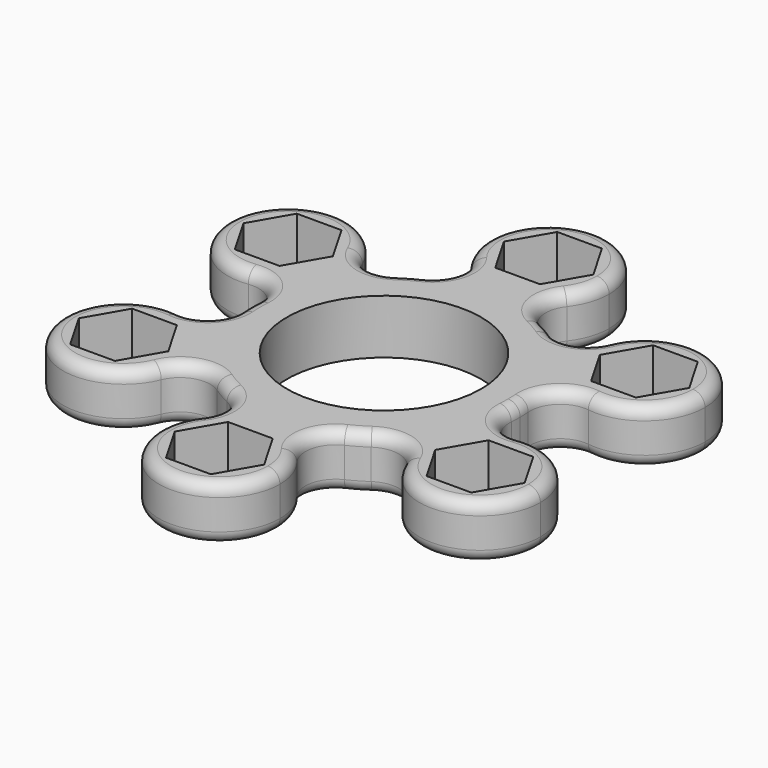
from build123d import *

# Parameters (mm, degrees)
F0_R     = 16.05
F1_DEPTH = 9
F2_R     = 2


# Not quite as in the source:
# - a feature names something its author has since deleted; it is built from what else it names


with BuildPart() as f1:
    # F0 (on Top) → F1 (new body)
    with BuildSketch(Plane.XY):
        with BuildLine():
            ThreePointArc((22.4319147865, -1.749056606), (22.4829722534, -0.8751906374), (22.5, 0))
            ThreePointArc((22.5, 0), (22.4829722534, 0.8751906374), (22.4319147865, 1.749056606))
            ThreePointArc((22.4319147865, 1.749056606), (19.4855715851, 11.25), (12.7306848467, 18.5520797576))
            ThreePointArc((12.7306848467, 18.5520797576), (11.25, 19.4855715851), (9.7012299398, 20.3011363636))
            ThreePointArc((9.7012299398, 20.3011363636), (0, 22.5), (-9.7012299398, 20.3011363636))
            ThreePointArc((-9.7012299398, 20.3011363636), (-11.25, 19.4855715851), (-12.7306848467, 18.5520797576))
            ThreePointArc((-12.7306848467, 18.5520797576), (-19.4855715851, 11.25), (-22.4319147865, 1.749056606))
            ThreePointArc((-22.4319147865, 1.749056606), (-22.5, 0), (-22.4319147865, -1.749056606))
            ThreePointArc((-22.4319147865, -1.749056606), (-19.4855715851, -11.25), (-12.7306848467, -18.5520797576))
            ThreePointArc((-12.7306848467, -18.5520797576), (-11.25, -19.4855715851), (-9.7012299398, -20.3011363636))
            ThreePointArc((-9.7012299398, -20.3011363636), (0, -22.5), (9.7012299398, -20.3011363636))
            ThreePointArc((9.7012299398, -20.3011363636), (11.25, -19.4855715851), (12.7306848467, -18.5520797576))
            ThreePointArc((12.7306848467, -18.5520797576), (19.4855715851, -11.25), (22.4319147865, -1.749056606))
        make_face()
        Circle(F0_R, mode=Mode.SUBTRACT)
        with BuildLine():
            ThreePointArc((12.7306848467, 18.5520797576), (19.4855715851, 11.25), (22.4319147865, 1.749056606))
            ThreePointArc((22.4319147865, 1.749056606), (23.9849013008, 5.7739668766), (28.0928110689, 7.0918239012))
            ThreePointArc((28.0928110689, 7.0918239012), (20.7846096908, 12), (20.1881051921, 20.7831760988))
            ThreePointArc((20.1881051921, 20.7831760988), (16.9928526462, 17.8845503954), (12.7306848467, 18.5520797576))
        make_face()
        with BuildLine():
            ThreePointArc((28.0928110689, -7.0918239012), (23.9849013008, -5.7739668766), (22.4319147865, -1.749056606))
            ThreePointArc((22.4319147865, -1.749056606), (19.4855715851, -11.25), (12.7306848467, -18.5520797576))
            ThreePointArc((12.7306848467, -18.5520797576), (16.9928526462, -17.8845503954), (20.1881051921, -20.7831760988))
            ThreePointArc((20.1881051921, -20.7831760988), (20.7846096908, -12), (28.0928110689, -7.0918239012))
        make_face()
        with BuildLine():
            ThreePointArc((20.1881051921, 20.7831760988), (20.7846096908, 12), (28.0928110689, 7.0918239012))
            ThreePointArc((28.0928110689, 7.0918239012), (36.0205565972, 9.4660592451), (39.4448637287, 17))
            ThreePointArc((39.4448637287, 17), (31.3726104228, 26.8124305186), (20.1881051921, 20.7831760988))
        make_face()
        Polygon((36.8349471743, 17), (33.1399054515, 10.6), (25.7498220059, 10.6), (22.054780283, 17), (25.7498220059, 23.4), (33.1399054515, 23.4), align=None, mode=Mode.SUBTRACT)
        with BuildLine():
            ThreePointArc((39.4448637287, -17), (36.0205565972, -9.4660592451), (28.0928110689, -7.0918239012))
            ThreePointArc((28.0928110689, -7.0918239012), (20.7846096908, -12), (20.1881051921, -20.7831760988))
            ThreePointArc((20.1881051921, -20.7831760988), (31.3726104228, -26.8124305186), (39.4448637287, -17))
        make_face()
        Polygon((22.054780283, -17), (25.7498220059, -10.6), (33.1399054515, -10.6), (36.8349471743, -17), (33.1399054515, -23.4), (25.7498220059, -23.4), align=None, mode=Mode.SUBTRACT)
        with BuildLine():
            ThreePointArc((-9.7012299398, 20.3011363636), (0, 22.5), (9.7012299398, 20.3011363636))
            ThreePointArc((9.7012299398, 20.3011363636), (6.9920486546, 23.6585172721), (7.9047058769, 27.875))
            ThreePointArc((7.9047058769, 27.875), (0, 24), (-7.9047058769, 27.875))
            ThreePointArc((-7.9047058769, 27.875), (-6.9920486546, 23.6585172721), (-9.7012299398, 20.3011363636))
        make_face()
        with BuildLine():
            ThreePointArc((7.9047058769, -27.875), (6.9920486546, -23.6585172721), (9.7012299398, -20.3011363636))
            ThreePointArc((9.7012299398, -20.3011363636), (0, -22.5), (-9.7012299398, -20.3011363636))
            ThreePointArc((-9.7012299398, -20.3011363636), (-6.9920486546, -23.6585172721), (-7.9047058769, -27.875))
            ThreePointArc((-7.9047058769, -27.875), (0, -24), (7.9047058769, -27.875))
        make_face()
        with BuildLine():
            ThreePointArc((-7.9047058769, 27.875), (0, 24), (7.9047058769, 27.875))
            ThreePointArc((7.9047058769, 27.875), (9.4616874491, 30.7632623499), (10, 34))
            ThreePointArc((10, 34), (-3.2367376501, 43.4616874491), (-7.9047058769, 27.875))
        make_face()
        Polygon((7.3900834456, 34), (3.6950417228, 27.6), (-3.6950417228, 27.6), (-7.3900834456, 34), (-3.6950417228, 40.4), (3.6950417228, 40.4), align=None, mode=Mode.SUBTRACT)
        with BuildLine():
            ThreePointArc((10, -34), (9.4616874491, -30.7632623499), (7.9047058769, -27.875))
            ThreePointArc((7.9047058769, -27.875), (0, -24), (-7.9047058769, -27.875))
            ThreePointArc((-7.9047058769, -27.875), (-3.2367376501, -43.4616874491), (10, -34))
        make_face()
        Polygon((-7.3900834456, -34), (-3.6950417228, -27.6), (3.6950417228, -27.6), (7.3900834456, -34), (3.6950417228, -40.4), (-3.6950417228, -40.4), align=None, mode=Mode.SUBTRACT)
        with BuildLine():
            ThreePointArc((-22.4319147865, 1.749056606), (-19.4855715851, 11.25), (-12.7306848467, 18.5520797576))
            ThreePointArc((-12.7306848467, 18.5520797576), (-16.9928526462, 17.8845503954), (-20.1881051921, 20.7831760988))
            ThreePointArc((-20.1881051921, 20.7831760988), (-19.63243321, 18.9277466942), (-19.4448637287, 17))
            ThreePointArc((-19.4448637287, 17), (-21.9109229737, 10.4243071315), (-28.0928110689, 7.0918239012))
            ThreePointArc((-28.0928110689, 7.0918239012), (-23.9849013008, 5.7739668766), (-22.4319147865, 1.749056606))
        make_face()
        with BuildLine():
            ThreePointArc((-20.1881051921, -20.7831760988), (-16.9928526462, -17.8845503954), (-12.7306848467, -18.5520797576))
            ThreePointArc((-12.7306848467, -18.5520797576), (-19.4855715851, -11.25), (-22.4319147865, -1.749056606))
            ThreePointArc((-22.4319147865, -1.749056606), (-23.9849013008, -5.7739668766), (-28.0928110689, -7.0918239012))
            ThreePointArc((-28.0928110689, -7.0918239012), (-21.9109229737, -10.4243071315), (-19.4448637287, -17))
            ThreePointArc((-19.4448637287, -17), (-19.63243321, -18.9277466942), (-20.1881051921, -20.7831760988))
        make_face()
        with BuildLine():
            ThreePointArc((-19.4448637287, 17), (-19.63243321, 18.9277466942), (-20.1881051921, 20.7831760988))
            ThreePointArc((-20.1881051921, 20.7831760988), (-38.1051177665, 22), (-28.0928110689, 7.0918239012))
            ThreePointArc((-28.0928110689, 7.0918239012), (-21.9109229737, 10.4243071315), (-19.4448637287, 17))
        make_face()
        Polygon((-25.7498220059, 23.4), (-22.054780283, 17), (-25.7498220059, 10.6), (-33.1399054515, 10.6), (-36.8349471743, 17), (-33.1399054515, 23.4), align=None, mode=Mode.SUBTRACT)
        with BuildLine():
            ThreePointArc((-28.0928110689, -7.0918239012), (-38.1051177665, -22), (-20.1881051921, -20.7831760988))
            ThreePointArc((-20.1881051921, -20.7831760988), (-19.63243321, -18.9277466942), (-19.4448637287, -17))
            ThreePointArc((-19.4448637287, -17), (-21.9109229737, -10.4243071315), (-28.0928110689, -7.0918239012))
        make_face()
        Polygon((-33.1399054515, -10.6), (-25.7498220059, -10.6), (-22.054780283, -17), (-25.7498220059, -23.4), (-33.1399054515, -23.4), (-36.8349471743, -17), align=None, mode=Mode.SUBTRACT)
    extrude(amount=F1_DEPTH)

    # F2
    f2_edges = [f1.edges().sort_by_distance(p)[0] for p in [
        (-23.984901, 5.773967, 9),
        (-23.984901, 5.773967, 0),
    ]]
    fillet(f2_edges, radius=F2_R)


solid = f1.part
